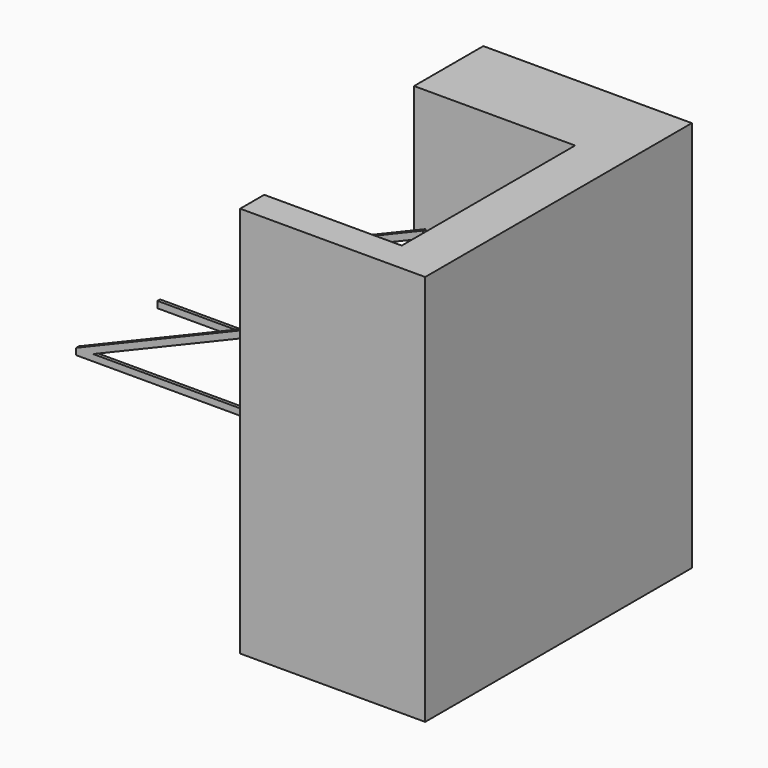
from build123d import *

# Parameters (mm, degrees)
F2_DEPTH  = 152.4
F3_W      = 1.27
F3_H      = 2.54
F4_DEPTH  = 126.6662840818
F8_DEPTH  = 1.27
F12_DEPTH = 1.27


# Not quite as in the source:
# - the program builds the solid bodies; features that only make, move or delete a surface that nothing else refers to are left out


with BuildPart() as f2:
    # F1 (on Top) → F2 (new body)
    with BuildSketch(Plane.XY):
        Polygon((-9.144, 0), (53.5142840818, 0), (53.5142840818, -84.328), (0, -84.328), (0, -96.0219023137), (53.5142840818, -96.0219023137), (71.9958739355, -96.0219023137), (71.9958739355, 33.6619690061), (53.5142840818, 33.6619690061), (-9.144, 33.6619690061), align=None)
    extrude(amount=F2_DEPTH)

    # F3 (on face) → F4 (join, through all)
    with BuildSketch(Plane(origin=(53.5142840818, 0, 0), x_dir=(0, -1, 0), z_dir=(-1, 0, 0))):
        with Locations((0.635, 74.93)):
            Rectangle(F3_W, F3_H)
        with Locations((83.693, 74.93)):
            Rectangle(F3_W, F3_H)
        with Locations((44.1576857662, 74.93)):
            Rectangle(F3_W, F3_H)
    extrude(amount=F4_DEPTH)

    # F7 (on face) → F8 (join)
    with BuildSketch(Plane.XZ):
        Polygon((-4.7359238379, 104.818597436), (-73.152, 76.2), (-66.5699955492, 76.2), (-4.7359238379, 102.0653302762), align=None)
    extrude(amount=F8_DEPTH)

    # F11 (on face) → F12 (join)
    with BuildSketch(Plane(origin=(0, -84.328, 0), x_dir=(-1, 0, 0), z_dir=(0, 1, 0))):
        Polygon((-5.7641793689, 106.457546895), (9.144, 100.221422174), (66.5699955492, 76.2), (73.152, 76.2), (9.144, 102.9746893338), (-5.7641793689, 109.2108140547), align=None)
    extrude(amount=F12_DEPTH)


solid = f2.part
